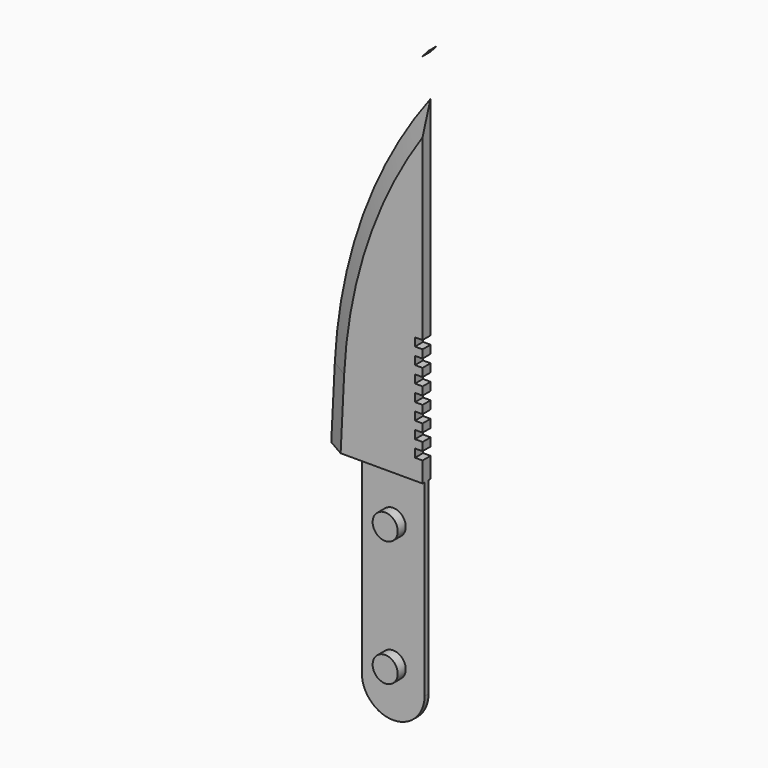
from build123d import *

# Parameters (mm, degrees)
F1_DEPTH    = 1.016
F3_DEPTH    = 0.508
F4_R        = 2.54
F5_DEPTH    = 2.032
F6_R        = 2.54
F7_DEPTH    = 2.032
F8_T1_DEPTH = 37.4993793655
F8_T4_ANGLE = 50.8590204833


# Not quite as in the source:
# - a fillet or chamfer that OpenCascade refuses, or shapes differently, is made with other operations: its cross-section is extruded or revolved along the edge and cut away or added


with BuildPart() as f1:
    # F0 (on Front) → F1 (new body, symmetric)
    with BuildSketch(Plane.XZ):
        with BuildLine():
            Line((1.2488319587, 64.6330847304), (0, 63.2437589053))
            Line((0, 63.2437589053), (0, 63.2175266339))
            ThreePointArc((0, 63.2175266339), (0.6211283352, 63.9282061037), (1.2488319587, 64.6330847304))
        make_face()
    extrude(amount=F1_DEPTH, both=True)


with BuildPart() as f1b:
    # F0 (on Front) → F1, piece 2 (new body, symmetric)
    with BuildSketch(Plane.XZ):
        with BuildLine():
            Line((0, 12.6442711507), (0, 63.2175266339))
            ThreePointArc((0, 63.2175266339), (-17.4739565434, 34.5701285719), (-24.6631958803, 1.793194445))
            Line((-24.6631958803, 1.793194445), (-25.4, -12.92445632))
            Line((-25.4, -12.92445632), (-20.955, -12.92445632))
            Line((-20.955, -12.92445632), (-4.445, -12.92445632))
            Line((-4.445, -12.92445632), (0, -12.92445632))
            Line((0, -12.92445632), (0, -8.8187288493))
            Line((0, -8.8187288493), (-1.524, -8.8187288493))
            Line((-1.524, -8.8187288493), (-1.524, -7.1677288493))
            Line((-1.524, -7.1677288493), (0, -7.1677288493))
            Line((0, -7.1677288493), (0, -5.5167288493))
            Line((0, -5.5167288493), (-1.524, -5.5167288493))
            Line((-1.524, -5.5167288493), (-1.524, -3.8657288493))
            Line((-1.524, -3.8657288493), (0, -3.8657288493))
            Line((0, -3.8657288493), (0, -2.2147288493))
            Line((0, -2.2147288493), (-1.524, -2.2147288493))
            Line((-1.524, -2.2147288493), (-1.524, -0.5637288493))
            Line((-1.524, -0.5637288493), (0, -0.5637288493))
            Line((0, -0.5637288493), (0, 1.0872711507))
            Line((0, 1.0872711507), (-1.524, 1.0872711507))
            Line((-1.524, 1.0872711507), (-1.524, 2.7382711507))
            Line((-1.524, 2.7382711507), (0, 2.7382711507))
            Line((0, 2.7382711507), (0, 4.3892711507))
            Line((0, 4.3892711507), (-1.524, 4.3892711507))
            Line((-1.524, 4.3892711507), (-1.524, 6.0402711507))
            Line((-1.524, 6.0402711507), (0, 6.0402711507))
            Line((0, 6.0402711507), (0, 7.6912711507))
            Line((0, 7.6912711507), (-1.524, 7.6912711507))
            Line((-1.524, 7.6912711507), (-1.524, 9.3422711507))
            Line((-1.524, 9.3422711507), (0, 9.3422711507))
            Line((0, 9.3422711507), (0, 10.9932711507))
            Line((0, 10.9932711507), (-1.524, 10.9932711507))
            Line((-1.524, 10.9932711507), (-1.524, 12.6442711507))
            Line((-1.524, 12.6442711507), (0, 12.6442711507))
        make_face()
    extrude(amount=F1_DEPTH, both=True)

    # F2 (on Front) → F3 (join, symmetric)
    with BuildSketch(Plane.XZ):
        with BuildLine():
            Line((0, -11.65445632), (-12.7, -11.65445632))
            Line((-12.7, -11.65445632), (-12.7, -51.02445632))
            ThreePointArc((-12.7, -51.02445632), (-10.8401280605, -55.5145843805), (-6.35, -57.37445632))
            ThreePointArc((-6.35, -57.37445632), (-1.8598719395, -55.5145843805), (0, -51.02445632))
            Line((0, -51.02445632), (0, -11.65445632))
        make_face()
    extrude(amount=F3_DEPTH, both=True)

    # F4 (on face) → F5 (join)
    with BuildSketch(Plane.XZ.offset(0.508)):
        with Locations((-6.35, -22.06845632)):
            Circle(F4_R)
        with Locations((-6.35, -47.46845632)):
            Circle(F4_R)
    extrude(amount=F5_DEPTH)

    # F6 (on face) → F7 (join)
    with BuildSketch(Plane(origin=(0, 0.508, 0), x_dir=(-1, 0, 0), z_dir=(0, 1, 0))):
        with Locations((6.35, -47.46845632)):
            Circle(F6_R)
        with Locations((6.35, -22.06845632)):
            Circle(F6_R)
    extrude(amount=F7_DEPTH)

    # F8: chamfer of 5.08 x 8.7988181024 on 1 edges, made by hand

    # F8_s2 → F8_t1 (cut)
    with BuildSketch(Plane(origin=(0.0278895878, 0, 0.5570940792), x_dir=(0, 1, 0), z_dir=(-0.05, 0, -0.9987492178))):
        Polygon((-1.016, -15.923189213), (4.064, -24.7220073154), (-1.016, -24.7220073154), align=None)
    extrude(amount=F8_T1_DEPTH, mode=Mode.SUBTRACT)

    # F8_s3 → F8_t4 (revolve, cut)
    with BuildSketch(Plane(origin=(48.3536933956, 0, 35.4868407309), x_dir=(0, 1, 0), z_dir=(0.8061865661, 0, 0.5916614071))):
        Polygon((-1.016, 44.7060536536), (4.064, 53.5048717561), (-1.016, 53.5048717561), align=None)
    revolve(axis=Axis((76.8097246454, -1.016, -3.286805555), (0, -1, 0)), revolution_arc=F8_T4_ANGLE, mode=Mode.SUBTRACT)


solid = Compound([f1.part, f1b.part])
